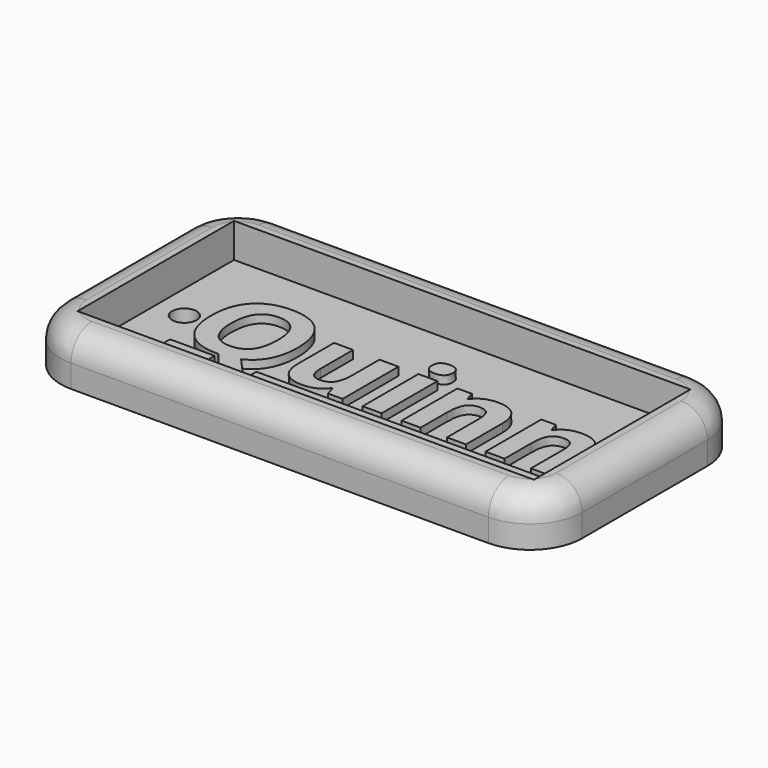
from build123d import *

# Parameters (mm, degrees)
F0_W         = 50.8
F0_H         = 25.4
F0_W_2       = 44.45
F0_H_2       = 19.05
F0_R         = 1.190625
F1_DEPTH     = 1.4111111111
F2_DEPTH     = 4.7625
F3_R         = 5.08
F4_T1_DEPTH  = 40.64
F4_T3_DEPTH  = 15.24
F4_T6_ANGLE  = 90
F4_T8_ANGLE  = 90
F4_T10_ANGLE = 90
F4_T12_ANGLE = 90
F5_W         = 4.3360870332
F5_H         = 1.0324008763
F5_W_2       = 27.9436726123
F5_H_2       = 1.0324013419
F5_TEXT_SIZE = 12.4414510944
F6_DEPTH     = 0.79375


# Not quite as in the source:
# - a fillet or chamfer that OpenCascade refuses, or shapes differently, is made with other operations: its cross-section is extruded or revolved along the edge and cut away or added
# - Text() gives the source's letters only with a copy of the font that has no kerning and outlines rounded to 1/6400 em; it was checked with that copy


with BuildPart() as f1:
    # F0 (on Top) → F1 (new body)
    with BuildSketch(Plane.XY):
        with Locations((25.4, 12.7)):
            Rectangle(F0_W, F0_H)
        with Locations((25.4, 12.7)):
            Rectangle(F0_W_2, F0_H_2, mode=Mode.SUBTRACT)
        with Locations((25.4, 12.7)):
            Rectangle(F0_W_2, F0_H_2)
        with Locations((5.953125, 12.7)):
            Circle(F0_R, mode=Mode.SUBTRACT)
    extrude(amount=F1_DEPTH)

    # F0 (on Top) → F2 (join)
    with BuildSketch(Plane.XY):
        with Locations((25.4, 12.7)):
            Rectangle(F0_W, F0_H)
        with Locations((25.4, 12.7)):
            Rectangle(F0_W_2, F0_H_2, mode=Mode.SUBTRACT)
    extrude(amount=F2_DEPTH)

    # F3
    f3_edges = [f1.edges().sort_by_distance(p)[0] for p in [
        (50.8, 0, 2.38125),
        (50.8, 25.4, 2.38125),
        (0, 25.4, 2.38125),
        (0, 0, 2.38125),
    ]]
    fillet(f3_edges, radius=F3_R)

    # F4: fillet of radius 2.54 on 8 edges, made by hand

    # F4_s2 → F4_t1 (cut)
    with BuildSketch(Plane.YZ.offset(5.08)):
        with BuildLine():
            ThreePointArc((2.54, 4.7625), (0.7439487758, 4.0185512242), (0, 2.2225))
            Line((0, 2.2225), (0, 4.7625))
            Line((0, 4.7625), (2.54, 4.7625))
        make_face()
        with BuildLine():
            ThreePointArc((22.86, 4.7625), (24.6560512242, 4.0185512242), (25.4, 2.2225))
            Line((25.4, 2.2225), (25.4, 4.7625))
            Line((25.4, 4.7625), (22.86, 4.7625))
        make_face()
    extrude(amount=F4_T1_DEPTH, mode=Mode.SUBTRACT)

    # F4_s4 → F4_t3 (cut)
    with BuildSketch(Plane.XZ.offset(-20.32)):
        with BuildLine():
            ThreePointArc((0, 2.2225), (0.7439487758, 4.0185512242), (2.54, 4.7625))
            Line((2.54, 4.7625), (0, 4.7625))
            Line((0, 4.7625), (0, 2.2225))
        make_face()
        with BuildLine():
            ThreePointArc((48.26, 4.7625), (50.0560512242, 4.0185512242), (50.8, 2.2225))
            Line((50.8, 2.2225), (50.8, 4.7625))
            Line((50.8, 4.7625), (48.26, 4.7625))
        make_face()
    extrude(amount=F4_T3_DEPTH, mode=Mode.SUBTRACT)

    # F4_s5 → F4_t6 (revolve, cut)
    with BuildSketch(Plane.XZ.offset(-20.32)):
        with BuildLine():
            ThreePointArc((2.54, 4.7625), (0.7439487758, 4.0185512242), (0, 2.2225))
            Line((0, 2.2225), (0, 4.7625))
            Line((0, 4.7625), (2.54, 4.7625))
        make_face()
    revolve(axis=Axis((5.08, 20.32, 4.7625), (0, 0, -1)), revolution_arc=F4_T6_ANGLE, mode=Mode.SUBTRACT)

    # F4_s7 → F4_t8 (revolve, cut)
    with BuildSketch(Plane.XZ.offset(-5.08)):
        with BuildLine():
            ThreePointArc((2.54, 4.7625), (0.7439487758, 4.0185512242), (0, 2.2225))
            Line((0, 2.2225), (0, 4.7625))
            Line((0, 4.7625), (2.54, 4.7625))
        make_face()
    revolve(axis=Axis((5.08, 5.08, 4.7625), (0, 0, 1)), revolution_arc=F4_T8_ANGLE, mode=Mode.SUBTRACT)

    # F4_s9 → F4_t10 (revolve, cut)
    with BuildSketch(Plane.XZ.offset(-20.32)):
        with BuildLine():
            ThreePointArc((48.26, 4.7625), (50.0560512242, 4.0185512242), (50.8, 2.2225))
            Line((50.8, 2.2225), (50.8, 4.7625))
            Line((50.8, 4.7625), (48.26, 4.7625))
        make_face()
    revolve(axis=Axis((45.72, 20.32, 4.7625), (0, 0, 1)), revolution_arc=F4_T10_ANGLE, mode=Mode.SUBTRACT)

    # F4_s11 → F4_t12 (revolve, cut)
    with BuildSketch(Plane.XZ.offset(-5.08)):
        with BuildLine():
            ThreePointArc((48.26, 4.7625), (50.0560512242, 4.0185512242), (50.8, 2.2225))
            Line((50.8, 2.2225), (50.8, 4.7625))
            Line((50.8, 4.7625), (48.26, 4.7625))
        make_face()
    revolve(axis=Axis((45.72, 5.08, 4.7625), (0, 0, -1)), revolution_arc=F4_T12_ANGLE, mode=Mode.SUBTRACT)

    # F5 (on face) → F6 (join)
    with BuildSketch(Plane.XY.offset(1.4111111111)):
        with Locations((10.6632038951, 7.2662341408)):
            Rectangle(F5_W, F5_H)
        with Locations((30.9326900169, 7.1974073071)):
            Rectangle(F5_W_2, F5_H_2)
        with Locations((7.7666573683, 8.3255321442)):
            Text('Quinn', F5_TEXT_SIZE, font='Open Sans', font_style=FontStyle.BOLD, text_align=(TextAlign.LEFT, TextAlign.BOTTOM))
    extrude(amount=F6_DEPTH)


solid = f1.part
